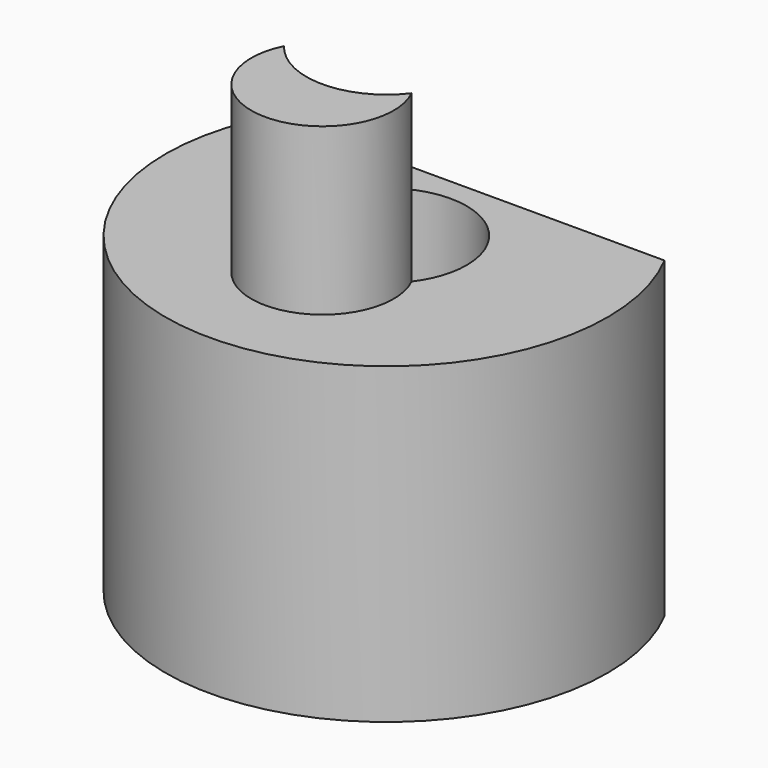
from build123d import *

# Parameters (mm, degrees)
F0_R     = 12
F1_DEPTH = 26
F2_R     = 12
F3_DEPTH = 9
F5_DEPTH = 15
F7_W     = 12
F7_H     = 17
F8_DEPTH = 6.425


with BuildPart() as f1:
    # F0 (on Top) → F1 (new body)
    with BuildSketch(Plane.XY):
        Circle(F0_R)
    extrude(amount=F1_DEPTH)

    # F2 (on face) → F3 (cut)
    with BuildSketch(Plane.XY.offset(26)):
        Circle(F2_R)
        with BuildLine():
            ThreePointArc((-3.462659053, -2.6329626437), (-1.3892323635, 4.1222000728), (4.35, 0))
            ThreePointArc((4.35, 0), (4.1222000728, -1.3892323635), (3.462659053, -2.6329626437))
            ThreePointArc((3.462659053, -2.6329626437), (0, -8.215), (-3.462659053, -2.6329626437))
        make_face(mode=Mode.SUBTRACT)
        with BuildLine():
            ThreePointArc((3.462659053, -2.6329626437), (4.1222000728, -1.3892323635), (4.35, 0))
            ThreePointArc((4.35, 0), (-1.3892323635, 4.1222000728), (-3.462659053, -2.6329626437))
            ThreePointArc((-3.462659053, -2.6329626437), (0, -4.35), (3.462659053, -2.6329626437))
        make_face()
    extrude(amount=-F3_DEPTH, mode=Mode.SUBTRACT)

    # F4 (on face) → F5 (cut)
    with BuildSketch(Plane.XY.offset(17)):
        with BuildLine():
            ThreePointArc((3.462659053, -2.6329626437), (4.1222000728, -1.3892323635), (4.35, 0))
            ThreePointArc((4.35, 0), (-1.3892323635, 4.1222000728), (-3.462659053, -2.6329626437))
            ThreePointArc((-3.462659053, -2.6329626437), (0, -4.35), (3.462659053, -2.6329626437))
        make_face()
    extrude(amount=-F5_DEPTH, mode=Mode.SUBTRACT)

    # F7 (on offset) → F8 (cut)
    with BuildSketch(Plane.XZ.offset(-12)):
        with Locations((6, 8.5)):
            Rectangle(F7_W, F7_H)
        with Locations((-6, 8.5)):
            Rectangle(F7_W, F7_H)
    extrude(amount=F8_DEPTH, mode=Mode.SUBTRACT)


solid = f1.part
